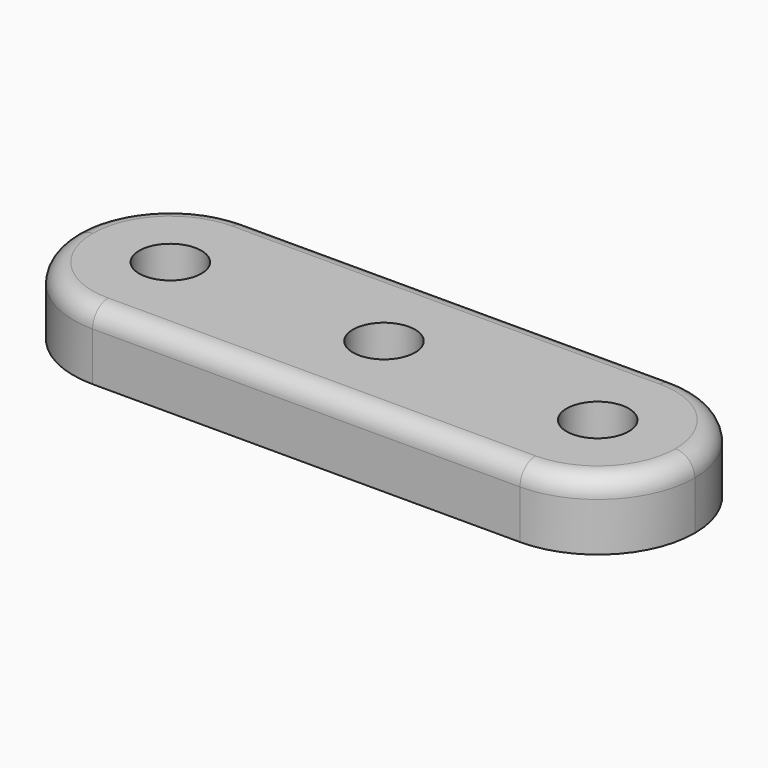
from build123d import *

# Parameters (mm, degrees)
F0_W     = 32
F0_H     = 10
F0_R     = 1.6
F1_DEPTH = 3.5
F2_R     = 4.99999
F3_R     = 1


# Not quite as in the source:
# - a fillet or chamfer is up to 0.001 mm smaller than in the source, because OpenCascade refuses the exact size


with BuildPart() as f1:
    # F0 (on Top) → F1 (new body)
    with BuildSketch(Plane.XY):
        with Locations((-9.4221055731, -0.7417218951)):
            Rectangle(F0_W, F0_H)
        with Locations((-20.4221047461, -0.7417218951)):
            Circle(F0_R, mode=Mode.SUBTRACT)
        with Locations((-9.4221055731, -0.7417218951)):
            Circle(F0_R, mode=Mode.SUBTRACT)
        with Locations((1.5778944269, -0.7417218951)):
            Circle(F0_R, mode=Mode.SUBTRACT)
    extrude(amount=F1_DEPTH)

    # F2 (radius 5 in the source; OpenCascade refuses exactly that, so slightly less here)
    f2_edges = [f1.edges().sort_by_distance(p)[0] for p in [
        (6.577894, 4.258278, 1.75),
        (6.577894, -5.741722, 1.75),
        (-25.422106, 4.258278, 1.75),
        (-25.422106, -5.741722, 1.75),
    ]]
    fillet(f2_edges, radius=F2_R)

    # F3
    f3_edges = [f1.edges().sort_by_distance(p)[0] for p in [
        (-9.422106, 4.258278, 3.5),
        (-9.422106, -5.741722, 3.5),
    ]]
    fillet(f3_edges, radius=F3_R)


solid = f1.part
